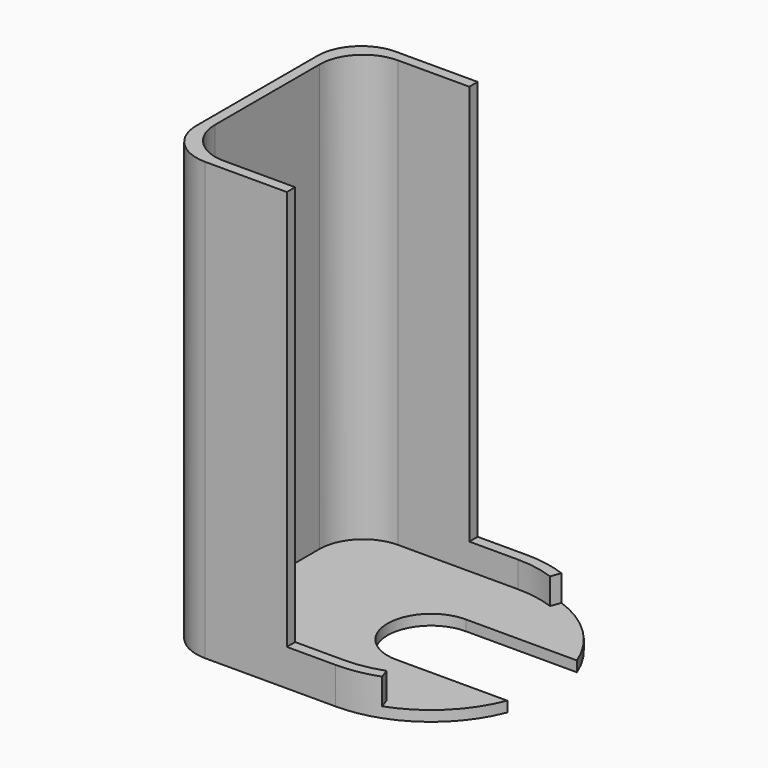
from build123d import *

# Parameters (mm, degrees)
F1_DEPTH = 1.2
F2_DEPTH = 49
F4_DEPTH = 46


# Not quite as in the source:
# - a feature names something its author has since deleted; it is built from what else it names


with BuildPart() as f1:
    # F0 (on Top) → F1 (new body)
    with BuildSketch(Plane.XY):
        with BuildLine():
            Line((-15, -13.7), (0, -13.7))
            ThreePointArc((0, -13.7), (2.378980034, -13.4918662163), (4.6856759636, -12.8737889048))
            Line((4.6856759636, -12.8737889048), (4.2752517916, -11.7461577598))
            ThreePointArc((4.2752517916, -11.7461577598), (2.1706022208, -12.3100969127), (0, -12.5))
            Line((0, -12.5), (-13.8, -12.5))
            ThreePointArc((-13.8, -12.5), (-17.3355339059, -11.0355339059), (-18.8, -7.5))
            Line((-18.8, -7.5), (-18.8, 7.5))
            ThreePointArc((-18.8, 7.5), (-17.3355339059, 11.0355339059), (-13.8, 12.5))
            Line((-13.8, 12.5), (0, 12.5))
            ThreePointArc((0, 12.5), (2.1706022208, 12.3100969127), (4.2752517916, 11.7461577598))
            Line((4.2752517916, 11.7461577598), (4.6856759636, 12.8737889048))
            ThreePointArc((4.6856759636, 12.8737889048), (2.378980034, 13.4918662163), (0, 13.7))
            Line((0, 13.7), (-15, 13.7))
            ThreePointArc((-15, 13.7), (-18.5355339059, 12.2355339059), (-20, 8.7))
            Line((-20, 8.7), (-20, -8.7))
            ThreePointArc((-20, -8.7), (-18.5355339059, -12.2355339059), (-15, -13.7))
        make_face()
        with BuildLine():
            Line((4.2752517916, -11.7461577598), (4.6856759636, -12.8737889048))
            ThreePointArc((4.6856759636, -12.8737889048), (9.5678327692, -9.8054360485), (12.75499902, -5))
            Line((12.75499902, -5), (11.4564392374, -5))
            ThreePointArc((11.4564392374, -5), (8.5585738758, -9.1104782099), (4.2752517916, -11.7461577598))
        make_face()
        with BuildLine():
            ThreePointArc((0, -12.5), (2.1706022208, -12.3100969127), (4.2752517916, -11.7461577598))
            ThreePointArc((4.2752517916, -11.7461577598), (8.5585738758, -9.1104782099), (11.4564392374, -5))
            Line((11.4564392374, -5), (0, -5))
            ThreePointArc((0, -5), (-5, 0), (0, 5))
            Line((0, 5), (11.4564392374, 5))
            ThreePointArc((11.4564392374, 5), (8.5585738758, 9.1104782099), (4.2752517916, 11.7461577598))
            ThreePointArc((4.2752517916, 11.7461577598), (2.1706022208, 12.3100969127), (0, 12.5))
            Line((0, 12.5), (-13.8, 12.5))
            ThreePointArc((-13.8, 12.5), (-17.3355339059, 11.0355339059), (-18.8, 7.5))
            Line((-18.8, 7.5), (-18.8, -7.5))
            ThreePointArc((-18.8, -7.5), (-17.3355339059, -11.0355339059), (-13.8, -12.5))
            Line((-13.8, -12.5), (0, -12.5))
        make_face()
        with BuildLine():
            ThreePointArc((4.2752517916, 11.7461577598), (8.5585738758, 9.1104782099), (11.4564392374, 5))
            Line((11.4564392374, 5), (12.75499902, 5))
            ThreePointArc((12.75499902, 5), (9.5678327692, 9.8054360485), (4.6856759636, 12.8737889048))
            Line((4.6856759636, 12.8737889048), (4.2752517916, 11.7461577598))
        make_face()
    extrude(amount=-F1_DEPTH)

    # F0 (on Top) → F2 (join)
    with BuildSketch(Plane.XY):
        with BuildLine():
            Line((-15, -13.7), (0, -13.7))
            ThreePointArc((0, -13.7), (2.378980034, -13.4918662163), (4.6856759636, -12.8737889048))
            Line((4.6856759636, -12.8737889048), (4.2752517916, -11.7461577598))
            ThreePointArc((4.2752517916, -11.7461577598), (2.1706022208, -12.3100969127), (0, -12.5))
            Line((0, -12.5), (-13.8, -12.5))
            ThreePointArc((-13.8, -12.5), (-17.3355339059, -11.0355339059), (-18.8, -7.5))
            Line((-18.8, -7.5), (-18.8, 7.5))
            ThreePointArc((-18.8, 7.5), (-17.3355339059, 11.0355339059), (-13.8, 12.5))
            Line((-13.8, 12.5), (0, 12.5))
            ThreePointArc((0, 12.5), (2.1706022208, 12.3100969127), (4.2752517916, 11.7461577598))
            Line((4.2752517916, 11.7461577598), (4.6856759636, 12.8737889048))
            ThreePointArc((4.6856759636, 12.8737889048), (2.378980034, 13.4918662163), (0, 13.7))
            Line((0, 13.7), (-15, 13.7))
            ThreePointArc((-15, 13.7), (-18.5355339059, 12.2355339059), (-20, 8.7))
            Line((-20, 8.7), (-20, -8.7))
            ThreePointArc((-20, -8.7), (-18.5355339059, -12.2355339059), (-15, -13.7))
        make_face()
    extrude(amount=F2_DEPTH)

    # F3 (on face) → F4 (cut)
    with BuildSketch(Plane.XY.offset(49)):
        with BuildLine():
            ThreePointArc((-5.6071383076, 12.5), (-2.8670542374, 13.3966413701), (0, 13.7))
            Line((0, 13.7), (-5.6071383076, 13.7))
            Line((-5.6071383076, 13.7), (-5.6071383076, 12.5))
        make_face()
        with BuildLine():
            Line((4.2752517916, 11.7461577598), (4.6856759636, 12.8737889048))
            ThreePointArc((4.6856759636, 12.8737889048), (2.378980034, 13.4918662163), (0, 13.7))
            ThreePointArc((0, 13.7), (-2.8670542374, 13.3966413701), (-5.6071383076, 12.5))
            Line((-5.6071383076, 12.5), (0, 12.5))
            ThreePointArc((0, 12.5), (2.1706022208, 12.3100969127), (4.2752517916, 11.7461577598))
        make_face()
        with BuildLine():
            ThreePointArc((0, -13.7), (2.378980034, -13.4918662163), (4.6856759636, -12.8737889048))
            Line((4.6856759636, -12.8737889048), (4.2752517916, -11.7461577598))
            ThreePointArc((4.2752517916, -11.7461577598), (2.1706022208, -12.3100969127), (0, -12.5))
            Line((0, -12.5), (-5.6071383076, -12.5))
            ThreePointArc((-5.6071383076, -12.5), (-2.8670542374, -13.3966413701), (0, -13.7))
        make_face()
        with BuildLine():
            Line((-5.6071383076, -13.7), (0, -13.7))
            ThreePointArc((0, -13.7), (-2.8670542374, -13.3966413701), (-5.6071383076, -12.5))
            Line((-5.6071383076, -12.5), (-5.6071383076, -13.7))
        make_face()
    extrude(amount=-F4_DEPTH, mode=Mode.SUBTRACT)


solid = f1.part
